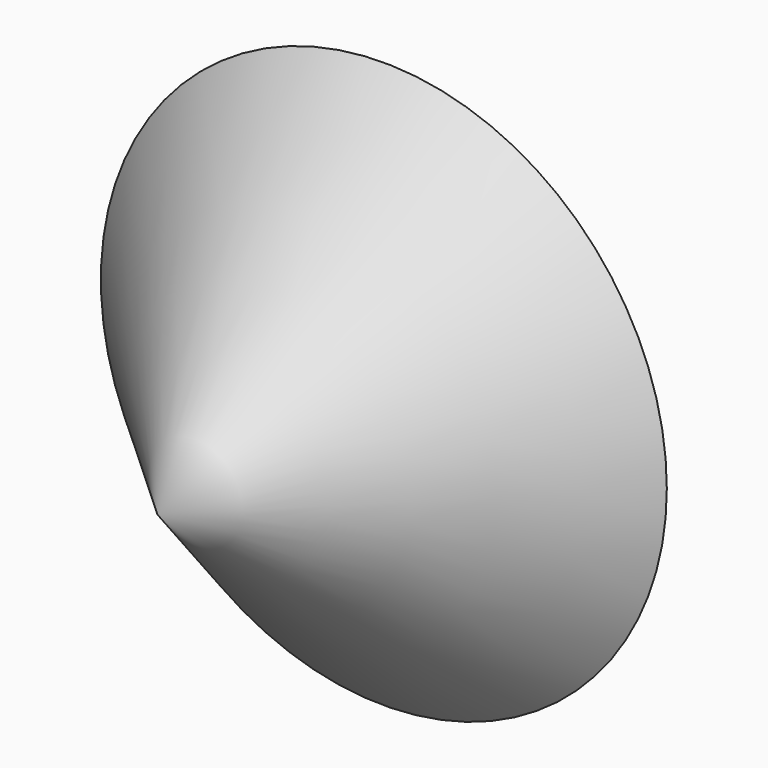
from build123d import *

# Parameters (mm, degrees)
F0_R = 51.4194692716


# Not quite as in the source:
# - an extrude whose draft closes it to a point is written as a loft to that point


with BuildPart() as f1:
    # F0 (on Front) → F1 section 0
    with BuildSketch(Plane.XZ, mode=Mode.PRIVATE) as f1_s0:
        with Locations((0, -2.1781306714)):
            Circle(F0_R)
    loft([f1_s0.sketch, Vertex(0, -51.4194692716, -2.1781306714)], ruled=True)


solid = f1.part
